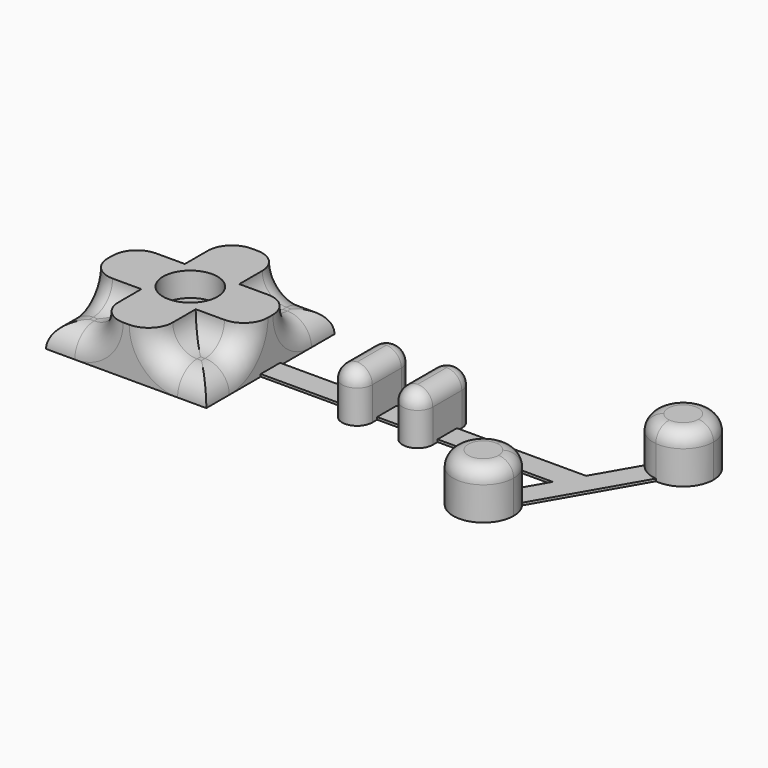
from build123d import *

# Parameters (mm, degrees)
F1_DEPTH = 8
F0_W     = 14.25
F0_H     = 4
F0_W_2   = 5
F2_DEPTH = 0.4
F3_R     = 2.49999
F4_R     = 4.5
F4_W     = 8.75
F4_H     = 8.75
F5_DEPTH = 4
F6_F1_R  = 3.9999
F6_F2_R  = 3.9999


# Not quite as in the source:
# - a fillet or chamfer is up to 0.001 mm smaller than in the source, because OpenCascade refuses the exact size


with BuildPart() as f1:
    # F0 (on Top) → F1 (new body)
    with BuildSketch(Plane.XY):
        Polygon((13.25, 2), (13.25, 13.25), (-13.25, 13.25), (-13.25, -13.25), (13.25, -13.25), (13.25, -2), align=None)
    extrude(amount=F1_DEPTH)



with BuildPart() as f1b:
    # F0 (on Top) → F1, piece 2 (new body)
    with BuildSketch(Plane.XY):
        Polygon((27.5, 3), (27.5, 2), (27.5, -2), (27.5, -3), (32.5, -3), (32.5, -2), (32.5, 2), (32.5, 3), align=None)
        with BuildLine():
            ThreePointArc((32.5, 3), (30, 5.5), (27.5, 3))
            Line((27.5, 3), (32.5, 3))
        make_face()
        with BuildLine():
            Line((32.5, -3), (27.5, -3))
            ThreePointArc((27.5, -3), (30, -5.5), (32.5, -3))
        make_face()
    extrude(amount=F1_DEPTH)


with BuildPart() as f1c:
    # F0 (on Top) → F1, piece 3 (new body)
    with BuildSketch(Plane.XY):
        with BuildLine():
            ThreePointArc((42.5, 3), (40, 5.5), (37.5, 3))
            Line((37.5, 3), (42.5, 3))
        make_face()
        Polygon((37.5, 3), (37.5, 2), (37.5, -2), (37.5, -3), (42.5, -3), (42.5, -2), (42.5, 2), (42.5, 3), align=None)
        with BuildLine():
            Line((42.5, -3), (37.5, -3))
            ThreePointArc((37.5, -3), (40, -5.5), (42.5, -3))
        make_face()
    extrude(amount=F1_DEPTH)


with BuildPart() as f1d:
    # F0 (on Top) → F1, piece 4 (new body)
    with BuildSketch(Plane.XY):
        with BuildLine():
            ThreePointArc((62.0951354248, -9.0313730334), (60.5717967697, -7.6698729811), (58.6310338096, -7.0313730334))
            ThreePointArc((58.6310338096, -7.0313730334), (54.3437822043, -15.3319524907), (63.0717967697, -12))
            ThreePointArc((63.0717967697, -12), (62.8213595536, -10.437420926), (62.0951354248, -9.0313730334))
        make_face()
    extrude(amount=F1_DEPTH)


with BuildPart() as f1e:
    # F0 (on Top) → F1, piece 5 (new body)
    with BuildSketch(Plane.XY):
        with BuildLine():
            ThreePointArc((76.9282032303, 12), (70.3656241563, 16.7495627838), (67.9048645752, 9.0313730334))
            ThreePointArc((67.9048645752, 9.0313730334), (69.4282032303, 7.6698729811), (71.3689661904, 7.0313730334))
            ThreePointArc((71.3689661904, 7.0313730334), (75.260155721, 8.2719854346), (76.9282032303, 12))
        make_face()
    extrude(amount=F1_DEPTH)


with BuildPart() as f1_1:
    add(f1.part)

    add(f1b.part)  # F2 merges F1b

    add(f1c.part)  # F2 merges F1c

    add(f1d.part)  # F2 merges F1d

    add(f1e.part)  # F2 merges F1e
    # F0 (on Top) → F2 (join)
    with BuildSketch(Plane.XY):
        with Locations((20.375, 0)):
            Rectangle(F0_W, F0_H)
        with Locations((35, 0)):
            Rectangle(F0_W_2, F0_H)
        Polygon((63.8452994616, 2), (42.5, 2), (42.5, -2), (61.5358983849, -2), align=None)
        with BuildLine():
            Line((67.9048645752, 9.0313730334), (63.8452994616, 2))
            Line((63.8452994616, 2), (61.5358983849, -2))
            Line((61.5358983849, -2), (58.6310338096, -7.0313730334))
            ThreePointArc((58.6310338096, -7.0313730334), (60.5717967697, -7.6698729811), (62.0951354248, -9.0313730334))
            Line((62.0951354248, -9.0313730334), (71.3689661904, 7.0313730334))
            ThreePointArc((71.3689661904, 7.0313730334), (69.4282032303, 7.6698729811), (67.9048645752, 9.0313730334))
        make_face()
    extrude(amount=F2_DEPTH)

    # F3 (radius 2.5 in the source; OpenCascade refuses exactly that, so slightly less here)
    f3_edges = [f1_1.edges().sort_by_distance(p)[0] for p in [
        (53.071797, -12, 8),
        (75.951542, 14.968627, 8),
        (42.5, 0, 8),
        (27.5, 0, 8),
        (30, -5.5, 8),
        (32.5, 0, 8),
        (30, 5.5, 8),
        (40, 5.5, 8),
        (37.5, 0, 8),
        (40, -5.5, 8),
    ]]
    fillet(f3_edges, radius=F3_R)

    # F4 (on face) → F5 (cut)
    with BuildSketch(Plane.XY.offset(8)):
        Circle(F4_R)
        with Locations((8.875, 8.875)):
            Rectangle(F4_W, F4_H)
        with Locations((-8.875, 8.875)):
            Rectangle(F4_W, F4_H)
        with Locations((-8.875, -8.875)):
            Rectangle(F4_W, F4_H)
        with Locations((8.875, -8.875)):
            Rectangle(F4_W, F4_H)
    extrude(amount=-F5_DEPTH, mode=Mode.SUBTRACT)

    # F6: fillet of radius 4 on 16 edges, made by hand

    # F6_f1 (radius 4 in the source; OpenCascade refuses exactly that, so slightly less here)
    f6_f1_edges = [f1_1.edges().sort_by_distance(p)[0] for p in [
        (-4.5, 8.875, 4),
        (-8.875, 4.5, 4),
        (4.5, 8.875, 4),
        (8.875, 4.5, 4),
        (-8.875, -4.5, 4),
        (-4.5, -8.875, 4),
        (8.875, -4.5, 4),
        (4.5, -8.875, 4),
    ]]
    fillet(f6_f1_edges, radius=F6_F1_R)

    # F6_f2 (radius 4 in the source; OpenCascade refuses exactly that, so slightly less here)
    f6_f2_edges = [f1_1.edges().sort_by_distance(p)[0] for p in [
        (-10.87495, 13.25, 4),
        (-13.25, 10.87495, 4),
        (13.25, 10.87495, 4),
        (10.87495, 13.25, 4),
        (-13.25, -10.87495, 4),
        (-10.87495, -13.25, 4),
        (13.25, -10.87495, 4),
        (10.87495, -13.25, 4),
        (5.6715435859, -13.25, 5.1715435859),
        (13.25, -5.6715435859, 5.1715435859),
        (-5.6715435859, -13.25, 5.1715435859),
        (-13.25, -5.6715435859, 5.1715435859),
        (5.6715435859, 13.25, 5.1715435859),
        (13.25, 5.6715435859, 5.1715435859),
        (-13.25, 5.6715435859, 5.1715435859),
        (-5.6715435859, 13.25, 5.1715435859),
    ]]
    fillet(f6_f2_edges, radius=F6_F2_R)


solid = f1_1.part
